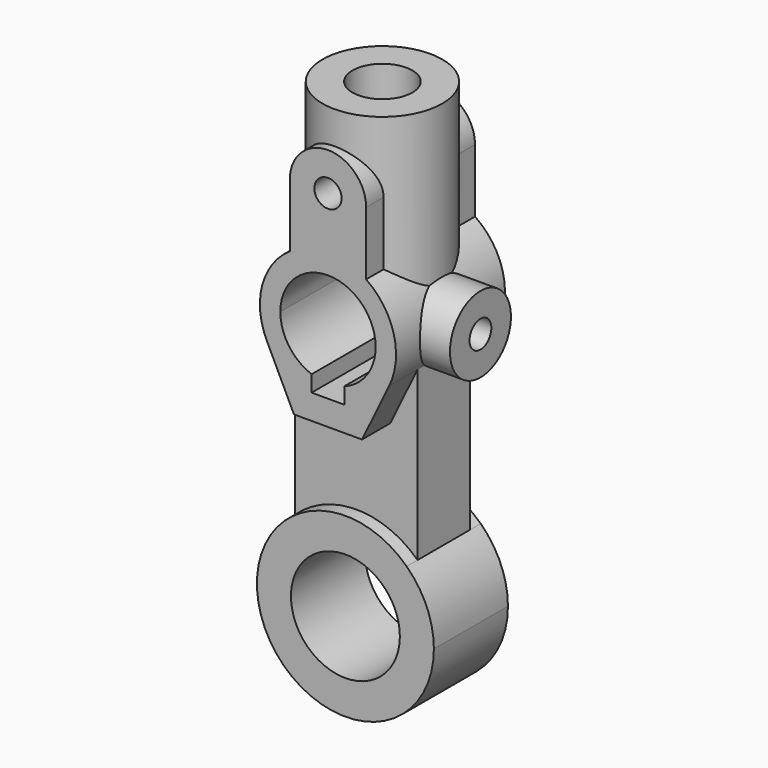
from build123d import *

# Parameters (mm, degrees)
F0_R          = 20
F1_DEPTH      = 17
F2_DEPTH      = 12
F0_R_2        = 5
F3_DEPTH      = 25
F5_R          = 14
F5_R_2        = 5
F7_END_RADIUS = 17.5
F7_REACH      = 82.643136
F9_R          = 22
F9_R_2        = 11
F11_REACH     = 229.613698


with BuildPart() as f1:
    # F0 (on Front) → F1 (new body, symmetric)
    with BuildSketch(Plane.XZ):
        with BuildLine():
            ThreePointArc((-22.5, 23.452079), (-12.747549, -29.895652), (32.5, 0))
            ThreePointArc((32.5, 0), (29.895652, 12.747549), (22.5, 23.452079))
            ThreePointArc((22.5, 23.452079), (0, 32.5), (-22.5, 23.452079))
        make_face()
        Circle(F0_R, mode=Mode.SUBTRACT)
    extrude(amount=F1_DEPTH, both=True)

    # F0 (on Front) → F2 (join, symmetric)
    with BuildSketch(Plane.XZ):
        with BuildLine():
            ThreePointArc((-22.5, 23.452079), (0, 32.5), (22.5, 23.452079))
            Line((22.5, 23.452079), (22.5, 85.102753))
            Line((22.5, 85.102753), (12.5, 64.455337))
            Line((12.5, 64.455337), (-12.5, 64.455337))
            Line((-12.5, 64.455337), (-22.5, 85.102753))
            Line((-22.5, 85.102753), (-22.5, 23.452079))
        make_face()
        with BuildLine():
            Line((12.5, 64.455337), (22.5, 85.102753))
            Line((22.5, 85.102753), (22.5, 96))
            Line((22.5, 96), (17.5, 96))
            ThreePointArc((17.5, 96), (14.33963, 85.968799), (6, 79.560718))
            Line((6, 79.560718), (6, 73.6))
            Line((6, 73.6), (-6, 73.6))
            Line((-6, 73.6), (-6, 79.560718))
            ThreePointArc((-6, 79.560718), (-14.33963, 85.968799), (-17.5, 96))
            Line((-17.5, 96), (-22.5, 96))
            Line((-22.5, 96), (-22.5, 85.102753))
            Line((-22.5, 85.102753), (-12.5, 64.455337))
            Line((-12.5, 64.455337), (12.5, 64.455337))
        make_face()
    extrude(amount=F2_DEPTH, both=True)

    # F0 (on Front) → F3 (join, symmetric)
    with BuildSketch(Plane.XZ):
        with BuildLine():
            Line((22.5, 96), (22.5, 85.102753))
            ThreePointArc((22.5, 85.102753), (24.142361, 102.492025), (14, 116.712315))
            ThreePointArc((14, 116.712315), (0, 121), (-14, 116.712315))
            ThreePointArc((-14, 116.712315), (-24.142361, 102.492025), (-22.5, 85.102753))
            Line((-22.5, 85.102753), (-22.5, 96))
            Line((-22.5, 96), (-17.5, 96))
            ThreePointArc((-17.5, 96), (0, 113.5), (17.5, 96))
            Line((17.5, 96), (22.5, 96))
        make_face()
        with BuildLine():
            Line((12.5, 64.455337), (22.5, 85.102753))
            Line((22.5, 85.102753), (22.5, 96))
            Line((22.5, 96), (17.5, 96))
            ThreePointArc((17.5, 96), (14.33963, 85.968799), (6, 79.560718))
            Line((6, 79.560718), (6, 73.6))
            Line((6, 73.6), (-6, 73.6))
            Line((-6, 73.6), (-6, 79.560718))
            ThreePointArc((-6, 79.560718), (-14.33963, 85.968799), (-17.5, 96))
            Line((-17.5, 96), (-22.5, 96))
            Line((-22.5, 96), (-22.5, 85.102753))
            Line((-22.5, 85.102753), (-12.5, 64.455337))
            Line((-12.5, 64.455337), (12.5, 64.455337))
        make_face()
        with BuildLine():
            ThreePointArc((-14, 116.712315), (0, 121), (14, 116.712315))
            Line((14, 116.712315), (14, 140))
            ThreePointArc((14, 140), (0, 154), (-14, 140))
            Line((-14, 140), (-14, 116.712315))
        make_face()
        with Locations((0, 140)):
            Circle(F0_R_2, mode=Mode.SUBTRACT)
    extrude(amount=F3_DEPTH, both=True)

    # F5 (on offset) → F6 (join, up to the next surface of F1)
    with BuildSketch(Plane.YZ.offset(36)):
        with Locations((0, 96)):
            Circle(F5_R)
        with Locations((0, 96)):
            Circle(F5_R_2, mode=Mode.SUBTRACT)
    extrude(until=Until.NEXT, dir=(-1, 0, 0))

    f7_end = (Plane(origin=(0, 0, 96), x_dir=(0, 0, -1), z_dir=(0, -1, 0)) * Cylinder(F7_END_RADIUS, 575.039856, mode=Mode.PRIVATE)).faces().sort_by_distance((0, 0, 113.5))[0]
    # F5 (on offset) → F7 (cut, up to the whole of a round face its end follows)
    with BuildSketch(Plane.YZ.offset(36)):
        with Locations((0, 96)):
            Circle(F5_R_2)
    f7_long = extrude(amount=-F7_REACH, mode=Mode.PRIVATE)
    add(split(f7_long, bisect_by=f7_end, keep=Keep.ALL, mode=Mode.PRIVATE).solids().sort_by_distance((36, 0, 96))[0], mode=Mode.SUBTRACT)

    # F9 (on offset) → F10 (join, up to the next surface of F1)
    with BuildSketch(Plane.XY.offset(166)):
        Circle(F9_R)
        Circle(F9_R_2, mode=Mode.SUBTRACT)
        Circle(F9_R_2)
    extrude(until=Until.NEXT, dir=(0, 0, -1))

    f11_end = f1.faces().sort_by_distance((0, 0, 113.5))[0]
    # F9 (on offset) → F11 (cut, up to a face of the model that its end follows)
    with BuildSketch(Plane.XY.offset(166)):
        Circle(F9_R_2)
    f11_long = extrude(amount=-F11_REACH, mode=Mode.PRIVATE)
    add(split(f11_long, bisect_by=f11_end, keep=Keep.BOTTOM, mode=Mode.PRIVATE), mode=Mode.SUBTRACT)


solid = f1.part
